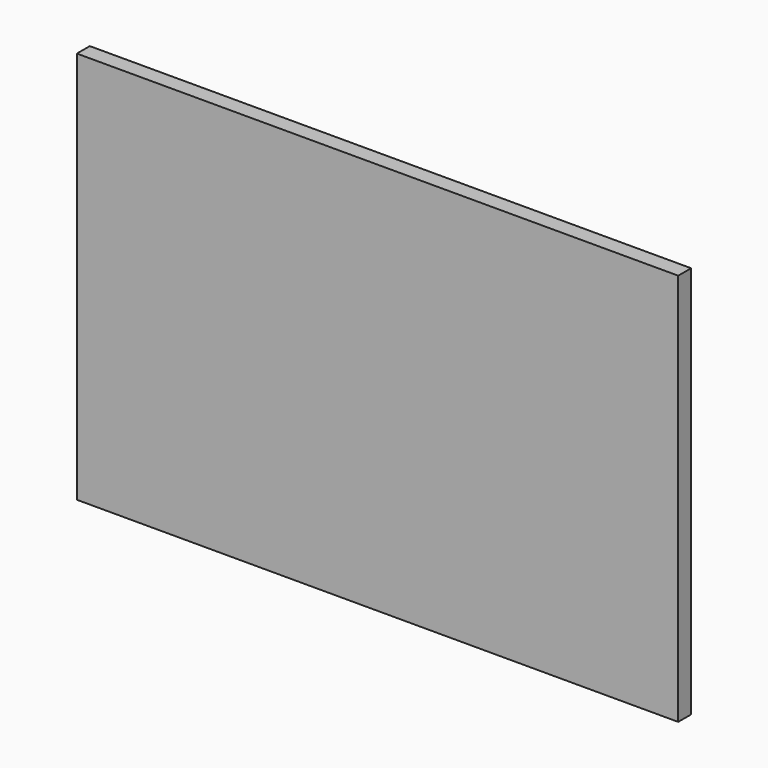
from build123d import *

# Parameters (mm, degrees)
F0_W     = 113.4197637439
F0_H     = 74.0887150168
F1_DEPTH = 3.048


# Not quite as in the source:
# - the program builds the solid bodies; features that only make, move or delete a surface that nothing else refers to are left out


with BuildPart() as f1:
    # F0 (on Front) → F1 (new body)
    with BuildSketch(Plane.XZ):
        Rectangle(F0_W, F0_H)
    extrude(amount=F1_DEPTH)


solid = f1.part
